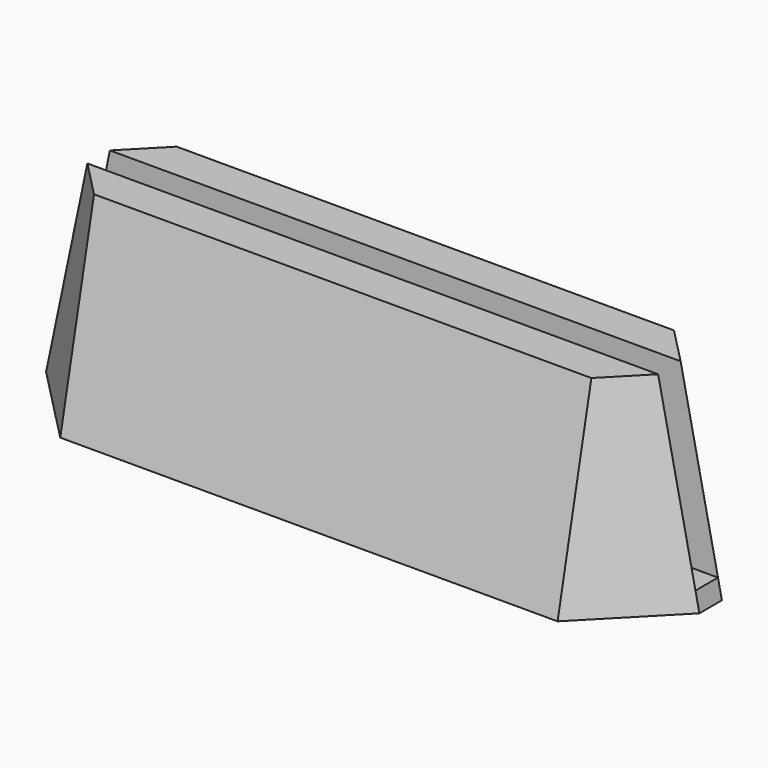
from build123d import *

# Parameters (mm, degrees)
F0_W        = 73
F0_H        = 20
F1_DEPTH    = 21
F2_W        = 3
F2_H        = 19
F3_DEPTH    = 73.001
F4_W        = 1.75
F4_H        = 3
F5_DEPTH    = 17
F6_R        = 1.74999
F7_T1_DEPTH = 72.9103913542
F7_T3_DEPTH = 72.9103913542
F9_DEPTH    = 20.001


# Not quite as in the source:
# - a fillet or chamfer that OpenCascade refuses, or shapes differently, is made with other operations: its cross-section is extruded or revolved along the edge and cut away or added
# - a fillet or chamfer is up to 0.001 mm smaller than in the source, because OpenCascade refuses the exact size


with BuildPart() as f1:
    # F0 (on Top) → F1 (new body)
    with BuildSketch(Plane.XY):
        with Locations((36.5, 10)):
            Rectangle(F0_W, F0_H)
    extrude(amount=F1_DEPTH)

    # F2 (on face) → F3 (cut, through all)
    with BuildSketch(Plane.YZ.offset(73)):
        Polygon((20, 21), (15.5, 21), (20, 0), align=None)
        with Locations((10, 11.5)):
            Rectangle(F2_W, F2_H)
        Polygon((4.5, 21), (0, 21), (0, 0), align=None)
    extrude(amount=-F3_DEPTH, mode=Mode.SUBTRACT)

    # F4 (on face) → F5 (join)
    with BuildSketch(Plane.XY.offset(2)):
        with Locations((35.625, 10)):
            Rectangle(F4_W, F4_H)
        with Locations((37.375, 10)):
            Rectangle(F4_W, F4_H)
    extrude(amount=F5_DEPTH)

    # F6 (radius 1.75 in the source; OpenCascade refuses exactly that, so slightly less here)
    f6_edges = [f1.edges().sort_by_distance(p)[0] for p in [
        (38.25, 10, 19),
        (34.75, 10, 19),
    ]]
    fillet(f6_edges, radius=F6_R)

    # F7: chamfer of 10 on 4 edges, made by hand

    # F7_s2 → F7_t1 (cut)
    with BuildSketch(Plane(origin=(0, -9.0103751492, 42.0484173631), x_dir=(1, 0, 0), z_dir=(0, 0.2095290887, -0.9778024141))):
        Polygon((73, -9.5560482815), (63, -19.5560482815), (73, -19.5560482815), align=None)
        Polygon((0, -9.5560482815), (10, -19.5560482815), (0, -19.5560482815), align=None)
    extrude(amount=F7_T1_DEPTH, mode=Mode.SUBTRACT)

    # F7_s4 → F7_t3 (cut)
    with BuildSketch(Plane(origin=(0, -5.3884239297, -25.1459783387), x_dir=(1, 0, 0), z_dir=(0, 0.2095290887, 0.9778024141))):
        Polygon((73, 10), (63, 0), (73, 0), align=None)
        Polygon((0, 10), (10, 0), (0, 0), align=None)
    extrude(amount=F7_T3_DEPTH, mode=Mode.SUBTRACT)

    # F8 (on Front) → F9 (cut, through all)
    with BuildSketch(Plane.XZ):
        Polygon((1.6886794803, 0), (6.0887903437, 21), (0, 21), (0, 0), align=None)
        Polygon((72.7780241408, 21), (66.9112096563, 21), (71.3113205197, 0), (72.7780241408, 0), align=None)
    extrude(amount=-F9_DEPTH, mode=Mode.SUBTRACT)


solid = f1.part
